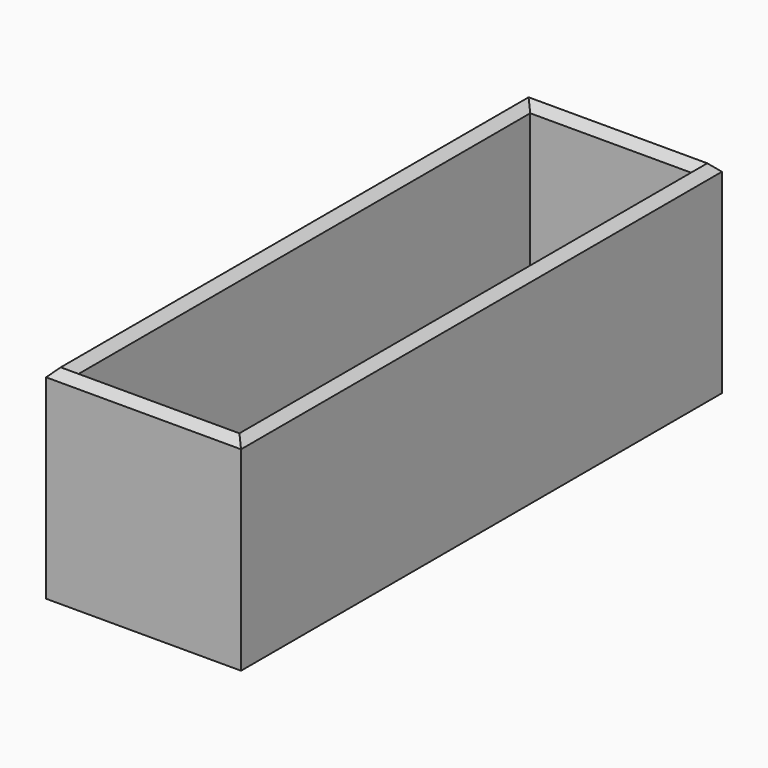
from build123d import *

# Parameters (mm, degrees)
F0_W     = 23.9999974624
F0_H     = 73.9999974624
F1_DEPTH = 25
F0_W_2   = 20
F0_H_2   = 6.8478258327
F2_DEPTH = 2.5
F3_SIZE  = 0.99999


# Not quite as in the source:
# - a fillet or chamfer is up to 0.001 mm smaller than in the source, because OpenCascade refuses the exact size


with BuildPart() as f1:
    # F0 (on Top) → F1 (new body)
    with BuildSketch(Plane.XY):
        with Locations((-2.6413043961, 7.5985620491)):
            Rectangle(F0_W, F0_H)
        Polygon((-12.6413043961, 12.7173913643), (-12.6413043961, 42.5985620491), (7.3586956039, 42.5985620491), (7.3586956039, 12.7173913643), (7.3586956039, 5.8695655316), (7.3586956039, -27.4014379509), (-12.6413043961, -27.4014379509), (-12.6413043961, 5.8695655316), align=None, mode=Mode.SUBTRACT)
    extrude(amount=F1_DEPTH)

    # F0 (on Top) → F2 (join)
    with BuildSketch(Plane.XY):
        with Locations((-2.6413043961, 7.5985620491)):
            Rectangle(F0_W, F0_H)
        Polygon((-12.6413043961, 12.7173913643), (-12.6413043961, 42.5985620491), (7.3586956039, 42.5985620491), (7.3586956039, 12.7173913643), (7.3586956039, 5.8695655316), (7.3586956039, -27.4014379509), (-12.6413043961, -27.4014379509), (-12.6413043961, 5.8695655316), align=None, mode=Mode.SUBTRACT)
        with Locations((-2.6413043961, 9.2934784479)):
            Rectangle(F0_W_2, F0_H_2)
    extrude(amount=F2_DEPTH)

    # F3 (size 1 in the source; OpenCascade refuses exactly that, so slightly less here)
    f3_edges = [f1.edges().sort_by_distance(p)[0] for p in [
        (-2.641304, -29.401437, 25),
        (-14.641303, 7.598562, 25),
        (9.358694, 7.598562, 25),
        (-2.641304, 44.598561, 25),
        (-2.641304, 42.598562, 25),
        (7.358696, 7.598562, 25),
        (-12.641304, 7.598562, 25),
        (-2.641304, -27.401438, 25),
    ]]
    chamfer(f3_edges, length=F3_SIZE)


solid = f1.part
